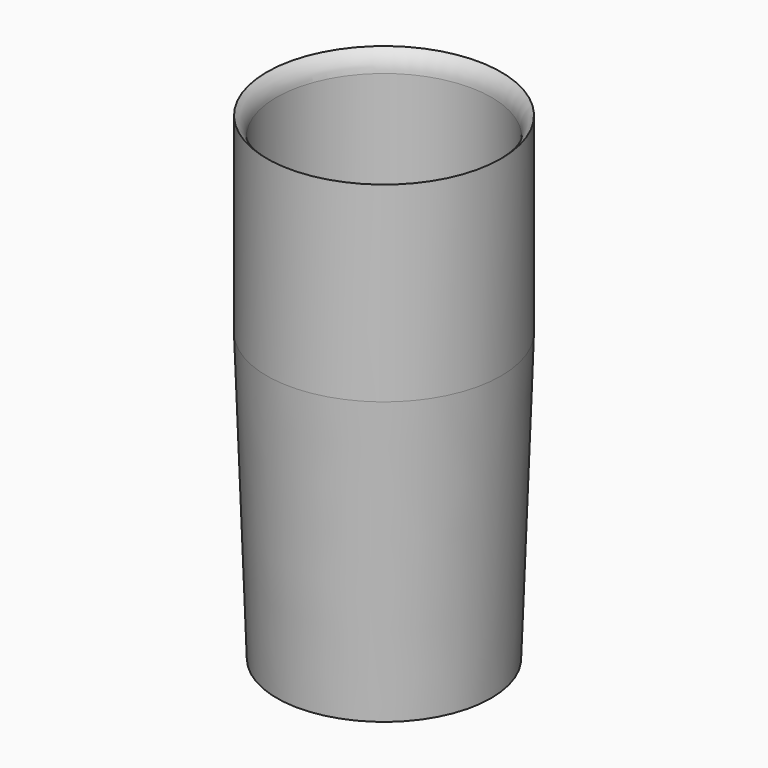
from build123d import *

# Parameters (mm, degrees)
F0_R          = 24.5
F1_DEPTH      = 70
F1_DEPTH_BACK = 30
F2_R          = 22.5
F3_DEPTH      = 81.3
F4_R          = 12
F5_DEPTH      = 41.2
F6_R          = 5
F7_SIZE2      = 2.0952461695
F7_SIZE       = 60


# Not quite as in the source:
# - a fillet or chamfer that OpenCascade refuses, or shapes differently, is made with other operations: its cross-section is extruded or revolved along the edge and cut away or added


with BuildPart() as f1:
    # F0 (on Top) → F1 (new body, two sides)
    with BuildSketch(Plane.XY) as f1_sk:
        Circle(F0_R)
    extrude(amount=F1_DEPTH)
    extrude(f1_sk.sketch, amount=-F1_DEPTH_BACK)

    # F2 (on Top) → F3 (cut)
    with BuildSketch(Plane.XY):
        Circle(F2_R)
    extrude(amount=F3_DEPTH, mode=Mode.SUBTRACT)

    # F4 (on Top) → F5 (cut)
    with BuildSketch(Plane.XY):
        Circle(F4_R)
    extrude(amount=-F5_DEPTH, mode=Mode.SUBTRACT)

    # F6
    f6_edges = [f1.edges().sort_by_distance(p)[0] for p in [
        (-12, 0, -30),
    ]]
    fillet(f6_edges, radius=F6_R)

    # F7
    f7_edges = [f1.edges().sort_by_distance(p)[0] for p in [
        (-24.5, 0, -30),
    ]]
    f7_side = f1.faces().sort_by_distance((-24.5, 0, -15))[0]
    chamfer(f7_edges, length=F7_SIZE, length2=F7_SIZE2, reference=f7_side)

    # F8: fillet of radius 5 on 1 edges, made by hand

    # F8_s1 → F8_t2 (revolve, cut)
    with BuildSketch(Plane.XZ):
        with BuildLine():
            ThreePointArc((24.5, 70), (23.027864045, 68.2360679775), (22.5, 66))
            Line((22.5, 66), (22.5, 70))
            Line((22.5, 70), (24.5, 70))
        make_face()
    revolve(axis=Axis((0, 0, 70), (0, 0, -1)), mode=Mode.SUBTRACT)


solid = f1.part
